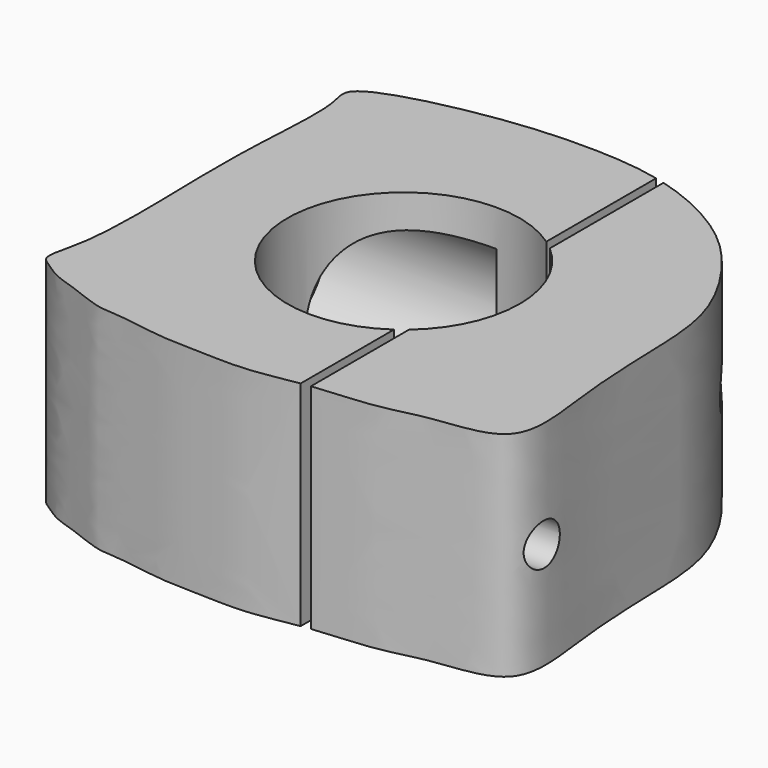
from build123d import *

# Parameters (mm, degrees)
F0_R     = 13.8079268521
F1_DEPTH = 25.4
F2_R     = 9.2981331684
F2_R_2   = 8.7836773463
F3_DEPTH = 26.3625290567
F5_D     = 5
F5_DEPTH = 30.542824105
F6_W     = 1.097727567
F6_H     = 54.2981084436
F7_DEPTH = 25.4010001


with BuildPart() as f1:
    # F0 (on Top) → F1 (new body)
    with BuildSketch(Plane.XY):
        with BuildLine():
            add(Edge.make_bspline(
                [(-26.2995827943, -20.1259739697), (-26.1594039772, -20.5785864069), (-25.2520524635, -21.1175272019), (-23.2996263658, -22.5482821093), (-20.6379874019, -23.2204020616), (-16.3721387177, -25.0875204997), (-13.9797594522, -24.9088487739), (-8.5740326759, -26.0033549278), (-3.8691621047, -25.9994806665), (2.5097478981, -26.3617816559), (8.6523499733, -24.8131266563), (16.3882818259, -24.6261545992), (21.6819049145, -22.7912826414), (31.7974099342, -22.4899972202), (29.6717484683, -10.6566994858), (29.2348805746, -0.1715888349), (29.034904765, 9.1137688251), (24.3219955961, 17.4440465585), (18.51954094, 23.5196401532), (9.278323197, 27.8552009151), (-0.3006060938, 28.7932495275), (-12.0270959879, 28.1780931863), (-26.4897184006, 24.5253193936), (-24.5911268233, 20.676159524), (-25.1308373128, 11.7651818458), (-25.519142472, 2.4798403845), (-24.7067948865, -14.5987374309), (-26.5646317144, -19.2701782068), (-26.2995827943, -20.1259739697)],
                knots=[0, 0, 0, 0, 0.0172467466, 0.0395191724, 0.0643276549, 0.0951163106, 0.1181042687, 0.1515024703, 0.1839518283, 0.2202086585, 0.2574004088, 0.2972167126, 0.3331203625, 0.3737027102, 0.4190172325, 0.4679834602, 0.5119237146, 0.5561043809, 0.5983501332, 0.6441039448, 0.6887053815, 0.7413226223, 0.7933842611, 0.8174343272, 0.8597167071, 0.9067176024, 0.9673899975, 1, 1, 1, 1], degree=3))
        make_face()
        Circle(F0_R, mode=Mode.SUBTRACT)
    extrude(amount=F1_DEPTH)

    # F2 (on Right) → F3 (cut, through all)
    with BuildSketch(Plane.YZ):
        with Locations((-10.924372822, 11.9697023183)):
            Circle(F2_R)
        with Locations((11.2106064335, 12.6580698416)):
            Circle(F2_R_2)
    extrude(amount=-F3_DEPTH, mode=Mode.SUBTRACT)

    # F5 (through all, one way)
    with BuildSketch(Plane(origin=(0, 0, 0), x_dir=(0, 1, 0), z_dir=(-1, 0, 0))):
        with Locations((-17.3108037561, -12.7176381648), (18.0163607001, -12.7176381648)):
            Circle(F5_D / 2)
    extrude(amount=-F5_DEPTH, mode=Mode.SUBTRACT)

    # F6 (on Top) → F7 (cut, through all)
    with BuildSketch(Plane.XY):
        with Locations((8.4646064788, 1.6199750826)):
            Rectangle(F6_W, F6_H)
    extrude(amount=F7_DEPTH, mode=Mode.SUBTRACT)


solid = f1.part
